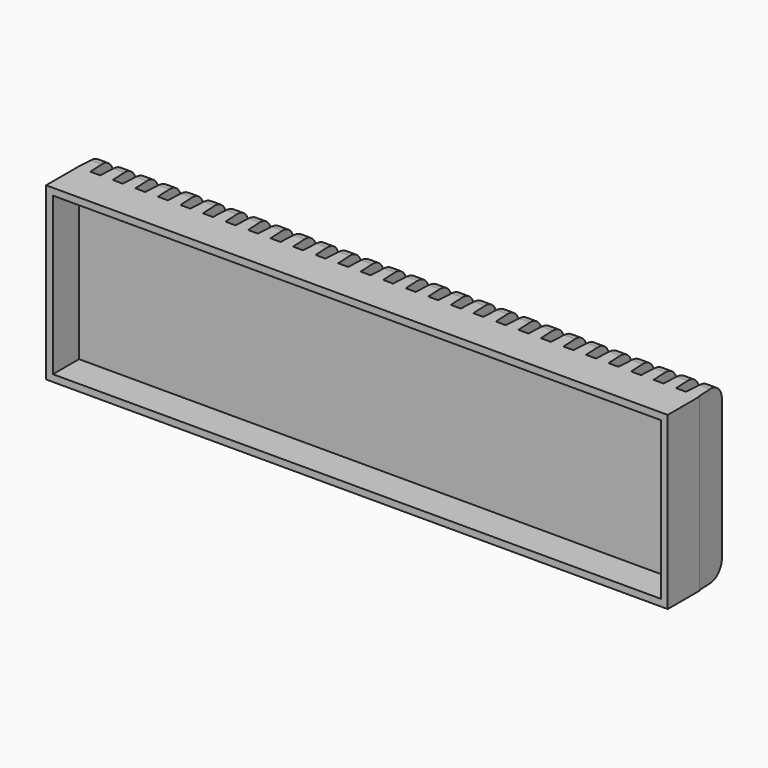
from build123d import *

# Parameters (mm, degrees)
F0_W        = 5080
F0_H        = 1397
F1_DEPTH    = 322.58
F3_DEPTH    = 1397
F4_T        = 55.88
F4_T3_DEPTH = 1508.76
F5_R        = 127


# Not quite as in the source:
# - a shell that OpenCascade refuses in one call is made with other operations: the cavity is built on its own and cut out


with BuildPart() as f1:
    # F0 (on Front) → F1 (new body)
    with BuildSketch(Plane.XZ):
        Rectangle(F0_W, F0_H)
    extrude(amount=F1_DEPTH)

    # F2 (on face) → F3 (join)
    with BuildSketch(Plane.XY.offset(698.5)):
        Polygon((-2526.6884240621, 254), (-2540, 0), (-2437.1768481242, 0), (-2450.4884240621, 254), align=None)
        Polygon((-2253.0268481242, 0), (-2266.3384240621, 254), (-2342.5384240621, 254), (-2355.85, 0), align=None)
        Polygon((-2068.8768481242, 0), (-2082.1884240621, 254), (-2158.3884240621, 254), (-2171.7, 0), align=None)
        Polygon((-1884.7268481242, 0), (-1898.0384240621, 254), (-1974.2384240621, 254), (-1987.55, 0), align=None)
        Polygon((-1700.5768481242, 0), (-1713.8884240621, 254), (-1790.0884240621, 254), (-1803.4, 0), align=None)
        Polygon((-1516.4268481242, 0), (-1529.7384240621, 254), (-1605.9384240621, 254), (-1619.25, 0), align=None)
        Polygon((-1332.2768481242, 0), (-1345.5884240621, 254), (-1421.7884240621, 254), (-1435.1, 0), align=None)
        Polygon((-1148.1268481242, 0), (-1161.4384240621, 254), (-1237.6384240621, 254), (-1250.95, 0), align=None)
        Polygon((-963.9768481242, 0), (-977.2884240621, 254), (-1053.4884240621, 254), (-1066.8, 0), align=None)
        Polygon((-779.8268481242, 0), (-793.1384240621, 254), (-869.3384240621, 254), (-882.65, 0), align=None)
        Polygon((-595.6768481242, 0), (-608.9884240621, 254), (-685.1884240621, 254), (-698.5, 0), align=None)
        Polygon((-411.5268481242, 0), (-424.8384240621, 254), (-501.0384240621, 254), (-514.35, 0), align=None)
        Polygon((-227.3768481242, 0), (-240.6884240621, 254), (-316.8884240621, 254), (-330.2, 0), align=None)
        Polygon((-43.2268481242, 0), (-56.5384240621, 254), (-132.7384240621, 254), (-146.05, 0), align=None)
        Polygon((140.9231518758, 0), (127.6115759379, 254), (51.4115759379, 254), (38.1, 0), align=None)
        Polygon((325.0731518758, 0), (311.7615759379, 254), (235.5615759379, 254), (222.25, 0), align=None)
        Polygon((509.2231518758, 0), (495.9115759379, 254), (419.7115759379, 254), (406.4, 0), align=None)
        Polygon((693.3731518758, 0), (680.0615759379, 254), (603.8615759379, 254), (590.55, 0), align=None)
        Polygon((877.5231518758, 0), (864.2115759379, 254), (788.0115759379, 254), (774.7, 0), align=None)
        Polygon((1061.6731518758, 0), (1048.3615759379, 254), (972.1615759379, 254), (958.85, 0), align=None)
        Polygon((1245.8231518758, 0), (1232.5115759379, 254), (1156.3115759379, 254), (1143, 0), align=None)
        Polygon((1429.9731518758, 0), (1416.6615759379, 254), (1340.4615759379, 254), (1327.15, 0), align=None)
        Polygon((1614.1231518758, 0), (1600.8115759379, 254), (1524.6115759379, 254), (1511.3, 0), align=None)
        Polygon((1798.2731518758, 0), (1784.9615759379, 254), (1708.7615759379, 254), (1695.45, 0), align=None)
        Polygon((1982.4231518758, 0), (1969.1115759379, 254), (1892.9115759379, 254), (1879.6, 0), align=None)
        Polygon((2166.5731518758, 0), (2153.2615759379, 254), (2077.0615759379, 254), (2063.75, 0), align=None)
        Polygon((2350.7231518758, 0), (2337.4115759379, 254), (2261.2115759379, 254), (2247.9, 0), align=None)
        Polygon((2534.8731518758, 0), (2521.5615759379, 254), (2445.3615759379, 254), (2432.05, 0), align=None)
    extrude(amount=-F3_DEPTH)

    # F4: shell of thickness 55.88, made by hand


with BuildPart() as f4_core1:
    # F4_t2: copy of F1
    add(f1.part)

    # the walls: a layer under each face that stays
    f4_faces = [f4_core1.faces().sort_by_distance(p)[0] for p in [
        (2540, -161.29, 0),
        (0, -34.29, -698.5),
        (0, -34.29, 698.5),
        (2537.4365759379, 0, 0),
        (-2540, -161.29, 0),
        (-2396.5134240621, 0, 0),
        (-2212.3634240621, 0, 0),
        (-2028.2134240621, 0, 0),
        (-1844.0634240621, 0, 0),
        (-1659.9134240621, 0, 0),
        (-1475.7634240621, 0, 0),
        (-1291.6134240621, 0, 0),
        (-1107.4634240621, 0, 0),
        (-923.3134240621, 0, 0),
        (-739.1634240621, 0, 0),
        (-555.0134240621, 0, 0),
        (-370.8634240621, 0, 0),
        (-186.7134240621, 0, 0),
        (-2.5634240621, 0, 0),
        (181.5865759379, 0, 0),
        (365.7365759379, 0, 0),
        (549.8865759379, 0, 0),
        (734.0365759379, 0, 0),
        (918.1865759379, 0, 0),
        (1102.3365759379, 0, 0),
        (1286.4865759379, 0, 0),
        (1470.6365759379, 0, 0),
        (1654.7865759379, 0, 0),
        (1838.9365759379, 0, 0),
        (2023.0865759379, 0, 0),
        (2207.2365759379, 0, 0),
        (2391.3865759379, 0, 0),
        (2528.2173639068, 127, 0),
        (-2533.3442120311, 127, 0),
        (-2443.8326360932, 127, 0),
        (-2488.5884240621, 254, 0),
        (-2349.1942120311, 127, 0),
        (-2259.6826360932, 127, 0),
        (-2304.4384240621, 254, 0),
        (-2165.0442120311, 127, 0),
        (-2075.5326360932, 127, 0),
        (-2120.2884240621, 254, 0),
        (-1980.8942120311, 127, 0),
        (-1891.3826360932, 127, 0),
        (-1936.1384240621, 254, 0),
        (-1796.7442120311, 127, 0),
        (-1707.2326360932, 127, 0),
        (-1751.9884240621, 254, 0),
        (-1612.5942120311, 127, 0),
        (-1523.0826360932, 127, 0),
        (-1567.8384240621, 254, 0),
        (-1428.4442120311, 127, 0),
        (-1338.9326360932, 127, 0),
        (-1383.6884240621, 254, 0),
        (-1244.2942120311, 127, 0),
        (-1154.7826360932, 127, 0),
        (-1199.5384240621, 254, 0),
        (-1060.1442120311, 127, 0),
        (-970.6326360932, 127, 0),
        (-1015.3884240621, 254, 0),
        (-875.9942120311, 127, 0),
        (-786.4826360932, 127, 0),
        (-831.2384240621, 254, 0),
        (-691.8442120311, 127, 0),
        (-602.3326360932, 127, 0),
        (-647.0884240621, 254, 0),
        (-507.6942120311, 127, 0),
        (-418.1826360932, 127, 0),
        (-462.9384240621, 254, 0),
        (-323.5442120311, 127, 0),
        (-234.0326360932, 127, 0),
        (-278.7884240621, 254, 0),
        (-139.3942120311, 127, 0),
        (-49.8826360932, 127, 0),
        (-94.6384240621, 254, 0),
        (44.7557879689, 127, 0),
        (134.2673639068, 127, 0),
        (89.5115759379, 254, 0),
        (228.9057879689, 127, 0),
        (318.4173639068, 127, 0),
        (273.6615759379, 254, 0),
        (413.0557879689, 127, 0),
        (502.5673639068, 127, 0),
        (457.8115759379, 254, 0),
        (597.2057879689, 127, 0),
        (686.7173639068, 127, 0),
        (641.9615759379, 254, 0),
        (781.3557879689, 127, 0),
        (870.8673639068, 127, 0),
        (826.1115759379, 254, 0),
        (965.5057879689, 127, 0),
        (1055.0173639068, 127, 0),
        (1010.2615759379, 254, 0),
        (1149.6557879689, 127, 0),
        (1239.1673639068, 127, 0),
        (1194.4115759379, 254, 0),
        (1333.8057879689, 127, 0),
        (1423.3173639068, 127, 0),
        (1378.5615759379, 254, 0),
        (1517.9557879689, 127, 0),
        (1607.4673639068, 127, 0),
        (1562.7115759379, 254, 0),
        (1702.1057879689, 127, 0),
        (1791.6173639068, 127, 0),
        (1746.8615759379, 254, 0),
        (1886.2557879689, 127, 0),
        (1975.7673639068, 127, 0),
        (1931.0115759379, 254, 0),
        (2070.4057879689, 127, 0),
        (2159.9173639068, 127, 0),
        (2115.1615759379, 254, 0),
        (2254.5557879689, 127, 0),
        (2344.0673639068, 127, 0),
        (2299.3115759379, 254, 0),
        (2438.7057879689, 127, 0),
        (2483.4615759379, 254, 0),
    ]]
    thicken(f4_faces, amount=-F4_T, mode=Mode.SUBTRACT)

    # F4_s4 → F4_t3 (cut)
    with BuildSketch(Plane.XY.offset(-754.38)):
        Polygon((2535.4311860598, 0.5880453323), (2534.8731518758, -55.88), (2481.8450118878, -55.88), (2479.0697334737, -2.9245332349), align=None)
        Polygon((-2436.6188139402, 0.5880453323), (-2437.1768481242, -55.88), (-2490.2049881122, -55.88), (-2492.9802665263, -2.9245332349), align=None)
        Polygon((-2356.408034184, 0.5880453323), (-2355.85, -55.88), (-2302.821860012, -55.88), (-2300.0465815979, -2.9245332349), align=None)
        Polygon((-2252.4688139402, 0.5880453323), (-2253.0268481242, -55.88), (-2306.0549881122, -55.88), (-2308.8302665263, -2.9245332349), align=None)
        Polygon((-2172.258034184, 0.5880453323), (-2171.7, -55.88), (-2118.671860012, -55.88), (-2115.8965815979, -2.9245332349), align=None)
        Polygon((-2068.3188139402, 0.5880453323), (-2068.8768481242, -55.88), (-2121.9049881122, -55.88), (-2124.6802665263, -2.9245332349), align=None)
        Polygon((-1988.108034184, 0.5880453323), (-1987.55, -55.88), (-1934.521860012, -55.88), (-1931.7465815979, -2.9245332349), align=None)
        Polygon((-1884.1688139402, 0.5880453323), (-1884.7268481242, -55.88), (-1937.7549881122, -55.88), (-1940.5302665263, -2.9245332349), align=None)
        Polygon((-1803.958034184, 0.5880453323), (-1803.4, -55.88), (-1750.371860012, -55.88), (-1747.5965815979, -2.9245332349), align=None)
        Polygon((-1700.0188139402, 0.5880453323), (-1700.5768481242, -55.88), (-1753.6049881122, -55.88), (-1756.3802665263, -2.9245332349), align=None)
        Polygon((-1619.808034184, 0.5880453323), (-1619.25, -55.88), (-1566.221860012, -55.88), (-1563.4465815979, -2.9245332349), align=None)
        Polygon((-1515.8688139402, 0.5880453323), (-1516.4268481242, -55.88), (-1569.4549881122, -55.88), (-1572.2302665263, -2.9245332349), align=None)
        Polygon((-1435.658034184, 0.5880453323), (-1435.1, -55.88), (-1382.071860012, -55.88), (-1379.2965815979, -2.9245332349), align=None)
        Polygon((-1331.7188139402, 0.5880453323), (-1332.2768481242, -55.88), (-1385.3049881122, -55.88), (-1388.0802665263, -2.9245332349), align=None)
        Polygon((-1251.508034184, 0.5880453323), (-1250.95, -55.88), (-1197.921860012, -55.88), (-1195.1465815979, -2.9245332349), align=None)
        Polygon((-1147.5688139402, 0.5880453323), (-1148.1268481242, -55.88), (-1201.1549881122, -55.88), (-1203.9302665263, -2.9245332349), align=None)
        Polygon((-1067.358034184, 0.5880453323), (-1066.8, -55.88), (-1013.771860012, -55.88), (-1010.9965815979, -2.9245332349), align=None)
        Polygon((-963.4188139402, 0.5880453323), (-963.9768481242, -55.88), (-1017.0049881122, -55.88), (-1019.7802665263, -2.9245332349), align=None)
        Polygon((-883.208034184, 0.5880453323), (-882.65, -55.88), (-829.621860012, -55.88), (-826.8465815979, -2.9245332349), align=None)
        Polygon((-779.2688139402, 0.5880453323), (-779.8268481242, -55.88), (-832.8549881122, -55.88), (-835.6302665263, -2.9245332349), align=None)
        Polygon((-699.058034184, 0.5880453323), (-698.5, -55.88), (-645.471860012, -55.88), (-642.6965815979, -2.9245332349), align=None)
        Polygon((-595.1188139402, 0.5880453323), (-595.6768481242, -55.88), (-648.7049881122, -55.88), (-651.4802665263, -2.9245332349), align=None)
        Polygon((-514.908034184, 0.5880453323), (-514.35, -55.88), (-461.321860012, -55.88), (-458.5465815979, -2.9245332349), align=None)
        Polygon((-410.9688139402, 0.5880453323), (-411.5268481242, -55.88), (-464.5549881122, -55.88), (-467.3302665263, -2.9245332349), align=None)
        Polygon((-330.758034184, 0.5880453323), (-330.2, -55.88), (-277.171860012, -55.88), (-274.3965815979, -2.9245332349), align=None)
        Polygon((-226.8188139402, 0.5880453323), (-227.3768481242, -55.88), (-280.4049881122, -55.88), (-283.1802665263, -2.9245332349), align=None)
        Polygon((-146.608034184, 0.5880453323), (-146.05, -55.88), (-93.021860012, -55.88), (-90.2465815979, -2.9245332349), align=None)
        Polygon((-42.6688139402, 0.5880453323), (-43.2268481242, -55.88), (-96.2549881122, -55.88), (-99.0302665263, -2.9245332349), align=None)
        Polygon((37.541965816, 0.5880453323), (38.1, -55.88), (91.128139988, -55.88), (93.9034184021, -2.9245332349), align=None)
        Polygon((141.4811860598, 0.5880453323), (140.9231518758, -55.88), (87.8950118878, -55.88), (85.1197334737, -2.9245332349), align=None)
        Polygon((221.691965816, 0.5880453323), (222.25, -55.88), (275.278139988, -55.88), (278.0534184021, -2.9245332349), align=None)
        Polygon((325.6311860598, 0.5880453323), (325.0731518758, -55.88), (272.0450118878, -55.88), (269.2697334737, -2.9245332349), align=None)
        Polygon((405.841965816, 0.5880453323), (406.4, -55.88), (459.428139988, -55.88), (462.2034184021, -2.9245332349), align=None)
        Polygon((509.7811860598, 0.5880453323), (509.2231518758, -55.88), (456.1950118878, -55.88), (453.4197334737, -2.9245332349), align=None)
        Polygon((589.991965816, 0.5880453323), (590.55, -55.88), (643.578139988, -55.88), (646.3534184021, -2.9245332349), align=None)
        Polygon((693.9311860598, 0.5880453323), (693.3731518758, -55.88), (640.3450118878, -55.88), (637.5697334737, -2.9245332349), align=None)
        Polygon((774.141965816, 0.5880453323), (774.7, -55.88), (827.728139988, -55.88), (830.5034184021, -2.9245332349), align=None)
        Polygon((878.0811860598, 0.5880453323), (877.5231518758, -55.88), (824.4950118878, -55.88), (821.7197334737, -2.9245332349), align=None)
        Polygon((958.291965816, 0.5880453323), (958.85, -55.88), (1011.878139988, -55.88), (1014.6534184021, -2.9245332349), align=None)
        Polygon((1062.2311860598, 0.5880453323), (1061.6731518758, -55.88), (1008.6450118878, -55.88), (1005.8697334737, -2.9245332349), align=None)
        Polygon((1142.441965816, 0.5880453323), (1143, -55.88), (1196.028139988, -55.88), (1198.8034184021, -2.9245332349), align=None)
        Polygon((1246.3811860598, 0.5880453323), (1245.8231518758, -55.88), (1192.7950118878, -55.88), (1190.0197334737, -2.9245332349), align=None)
        Polygon((1326.591965816, 0.5880453323), (1327.15, -55.88), (1380.178139988, -55.88), (1382.9534184021, -2.9245332349), align=None)
        Polygon((1430.5311860598, 0.5880453323), (1429.9731518758, -55.88), (1376.9450118878, -55.88), (1374.1697334737, -2.9245332349), align=None)
        Polygon((1510.741965816, 0.5880453323), (1511.3, -55.88), (1564.328139988, -55.88), (1567.1034184021, -2.9245332349), align=None)
        Polygon((1614.6811860598, 0.5880453323), (1614.1231518758, -55.88), (1561.0950118878, -55.88), (1558.3197334737, -2.9245332349), align=None)
        Polygon((1694.891965816, 0.5880453323), (1695.45, -55.88), (1748.478139988, -55.88), (1751.2534184021, -2.9245332349), align=None)
        Polygon((1798.8311860598, 0.5880453323), (1798.2731518758, -55.88), (1745.2450118878, -55.88), (1742.4697334737, -2.9245332349), align=None)
        Polygon((1879.041965816, 0.5880453323), (1879.6, -55.88), (1932.628139988, -55.88), (1935.4034184021, -2.9245332349), align=None)
        Polygon((1982.9811860598, 0.5880453323), (1982.4231518758, -55.88), (1929.3950118878, -55.88), (1926.6197334737, -2.9245332349), align=None)
        Polygon((2063.191965816, 0.5880453323), (2063.75, -55.88), (2116.778139988, -55.88), (2119.5534184021, -2.9245332349), align=None)
        Polygon((2167.1311860598, 0.5880453323), (2166.5731518758, -55.88), (2113.5450118878, -55.88), (2110.7697334737, -2.9245332349), align=None)
        Polygon((2247.341965816, 0.5880453323), (2247.9, -55.88), (2300.928139988, -55.88), (2303.7034184021, -2.9245332349), align=None)
        Polygon((2351.2811860598, 0.5880453323), (2350.7231518758, -55.88), (2297.6950118878, -55.88), (2294.9197334737, -2.9245332349), align=None)
        Polygon((2431.491965816, 0.5880453323), (2432.05, -55.88), (2485.078139988, -55.88), (2487.8534184021, -2.9245332349), align=None)
    extrude(amount=F4_T3_DEPTH, mode=Mode.SUBTRACT)


with BuildPart() as f1_1:
    add(f1.part)

    # what is left inside the walls is the cavity
    f4_cavity = [f4_core1.part.solids().sort_by_distance(p)[0] for p in [
        (0, -322.0212, -214.206667),
    ]]
    add(f4_cavity, mode=Mode.SUBTRACT)

    # F5
    f5_edges = [f1_1.edges().sort_by_distance(p)[0] for p in [
        (-2488.588424, 254, 698.5),
        (-2304.438424, 254, 698.5),
        (-2120.288424, 254, 698.5),
        (-1936.138424, 254, 698.5),
        (-1751.988424, 254, 698.5),
        (-1567.838424, 254, 698.5),
        (-1383.688424, 254, 698.5),
        (-1199.538424, 254, 698.5),
        (-1015.388424, 254, 698.5),
        (-831.238424, 254, 698.5),
        (-647.088424, 254, 698.5),
        (-462.938424, 254, 698.5),
        (-278.788424, 254, 698.5),
        (-94.638424, 254, 698.5),
        (89.511576, 254, 698.5),
        (273.661576, 254, 698.5),
        (457.811576, 254, 698.5),
        (641.961576, 254, 698.5),
        (826.111576, 254, 698.5),
        (1010.261576, 254, 698.5),
        (1194.411576, 254, 698.5),
        (1378.561576, 254, 698.5),
        (1562.711576, 254, 698.5),
        (1746.861576, 254, 698.5),
        (1931.011576, 254, 698.5),
        (2115.161576, 254, 698.5),
        (2299.311576, 254, 698.5),
        (2483.461576, 254, 698.5),
        (-2488.588424, 254, -698.5),
        (-2304.438424, 254, -698.5),
        (-2120.288424, 254, -698.5),
        (-1936.138424, 254, -698.5),
        (-1751.988424, 254, -698.5),
        (-1567.838424, 254, -698.5),
        (-1383.688424, 254, -698.5),
        (-1199.538424, 254, -698.5),
        (-1015.388424, 254, -698.5),
        (-831.238424, 254, -698.5),
        (-647.088424, 254, -698.5),
        (-462.938424, 254, -698.5),
        (-278.788424, 254, -698.5),
        (-94.638424, 254, -698.5),
        (89.511576, 254, -698.5),
        (273.661576, 254, -698.5),
        (457.811576, 254, -698.5),
        (641.961576, 254, -698.5),
        (826.111576, 254, -698.5),
        (1010.261576, 254, -698.5),
        (1194.411576, 254, -698.5),
        (1378.561576, 254, -698.5),
        (1562.711576, 254, -698.5),
        (1746.861576, 254, -698.5),
        (1931.011576, 254, -698.5),
        (2115.161576, 254, -698.5),
        (2299.311576, 254, -698.5),
        (2483.461576, 254, -698.5),
    ]]
    fillet(f5_edges, radius=F5_R)


solid = f1_1.part
